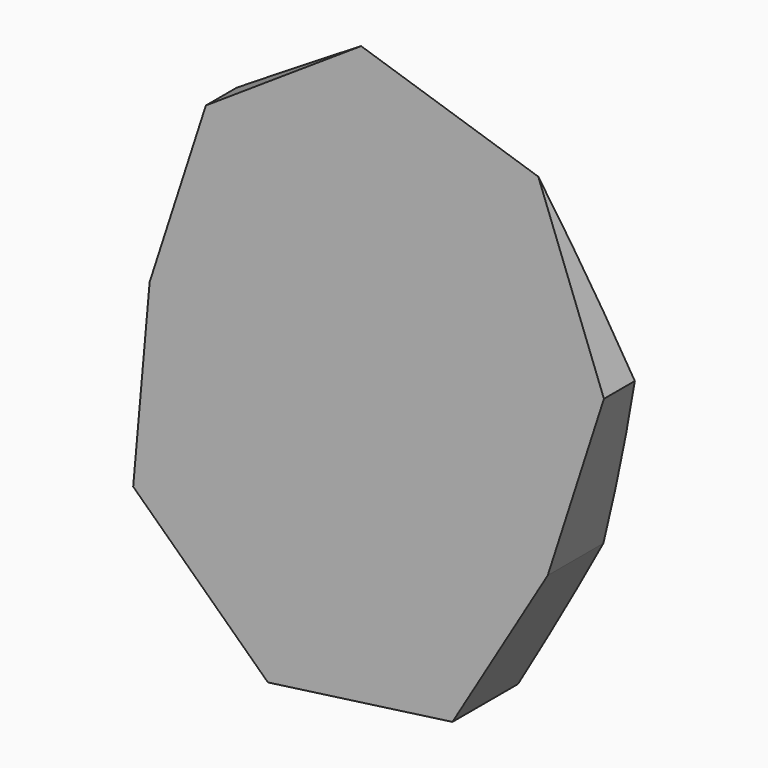
from build123d import *

# Parameters (mm, degrees)
F0_W        = 166.4632111788
F0_H        = 41.9475100935
F2_DEPTH    = 59.9997173995
F4_DEPTH    = 23.426502943
F5_DEPTH    = 103.8927901536
F6_T1_DEPTH = 1655.4987810503


# Not quite as in the source:
# - a fillet or chamfer that OpenCascade refuses, or shapes differently, is made with other operations: its cross-section is extruded or revolved along the edge and cut away or added


with BuildPart() as f2:
    # F0 (on Front) → F2 (new body)
    with BuildSketch(Plane.XZ):
        with Locations((185.5375096202, 20.9737550467)):
            Rectangle(F0_W, F0_H)
    extrude(amount=F2_DEPTH)


with BuildPart() as f4:
    # F3 (on offset) → F4 (new body, symmetric)
    with BuildSketch(Plane.XZ.offset(59.8023701459)):
        Polygon((304.9551667814, 11.8217294328), (267.6064548846, 110.9551588781), (166.814277799, 143.5634423701), (78.4772006558, 85.0918773514), (69.1148442917, -20.4292551163), (145.7772540063, -93.5403900459), (250.7360716562, -79.1873516402), align=None)
    extrude(amount=F4_DEPTH, both=True)

    # F5 (add): faces of the model
    f5_faces = [f4.faces().sort_by_distance(p)[0] for p in [
        (217.2103663418, -59.8023701459, 127.2593006241),
        (122.6457392274, -59.8023701459, 114.3276598607),
        (73.7960224737, -59.8023701459, 32.3313111175),
        (107.446049149, -59.8023701459, -56.9848225811),
        (198.2566628312, -59.8023701459, -86.3638708431),
        (277.8456192188, -59.8023701459, -33.6828111037),
        (286.280810833, -59.8023701459, 61.3884441555),
    ]]
    extrude(f5_faces, amount=F5_DEPTH, dir=(0.3078121651, 0, 0.9514471457))

    # F6: fillet of radius 1048.3963355256 on 3 edges, made by hand

    # F6_s2 → F6_t1 (cut)
    with BuildSketch(Plane(origin=(946.9197916988, 0, -306.3474756142), x_dir=(0, 1, 0), z_dir=(-0.9514471457, 0, 0.3078121651))):
        with BuildLine():
            ThreePointArc((-36.3758672029, 18.0793434638), (-48.1552934974, -138.6377897402), (-83.228873089, -291.833281639))
            Line((-83.228873089, -291.833281639), (-36.3758672029, -291.833281639))
            Line((-36.3758672029, -291.833281639), (-36.3758672029, 18.0793434638))
        make_face()
    extrude(amount=F6_T1_DEPTH, mode=Mode.SUBTRACT)


solid = Compound([f2.part, f4.part])
